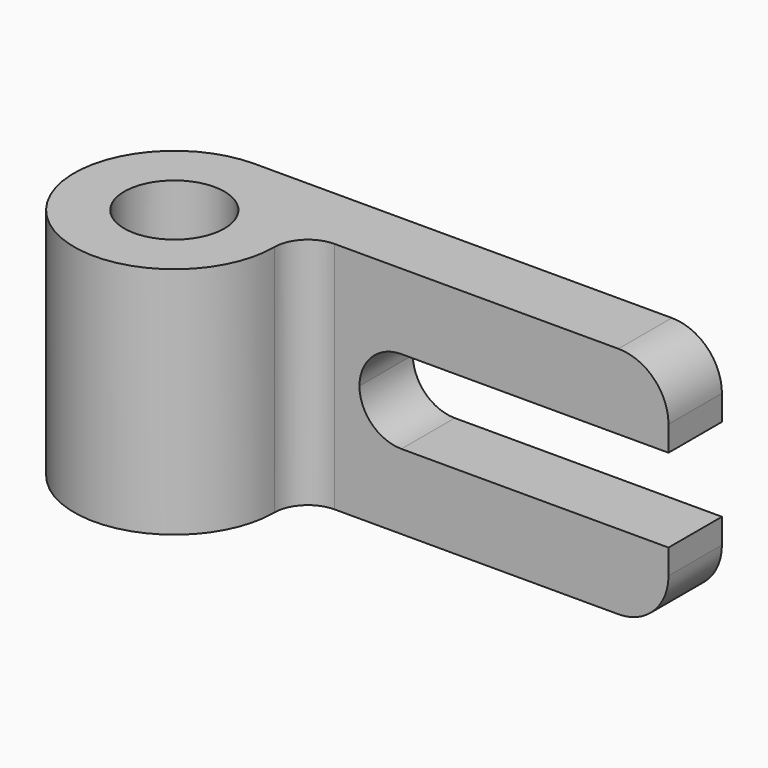
from build123d import *

# Parameters (mm, degrees)
F0_R        = 9.525
F1_DEPTH    = 44.45
F2_T1_DEPTH = 44.45
F3_R        = 9.525
F4_W        = 58.7756
F4_H        = 15.875
F5_DEPTH    = 25.4
F6_T1_DEPTH = 12.7


# Not quite as in the source:
# - a fillet or chamfer that OpenCascade refuses, or shapes differently, is made with other operations: its cross-section is extruded or revolved along the edge and cut away or added


with BuildPart() as f1:
    # F0 (on Top) → F1 (new body)
    with BuildSketch(Plane.XY):
        with BuildLine():
            ThreePointArc((0, 19.05), (10.9985226281, 15.5542598667), (17.9605122421, 6.35))
            Line((17.9605122421, 6.35), (88.9, 6.35))
            Line((88.9, 6.35), (88.9, 19.05))
            Line((88.9, 19.05), (0, 19.05))
        make_face()
        with BuildLine():
            ThreePointArc((0, 19.05), (-13.4703841816, -13.4703841816), (19.05, 0))
            ThreePointArc((19.05, 0), (18.7756525614, 3.2213926947), (17.9605122421, 6.35))
            ThreePointArc((17.9605122421, 6.35), (10.9985226281, 15.5542598667), (0, 19.05))
        make_face()
        Circle(F0_R, mode=Mode.SUBTRACT)
    extrude(amount=F1_DEPTH)

    # F2: fillet of radius 6.35 on 1 edges, made by hand

    # F2_s2 → F2_t1 (join)
    with BuildSketch(Plane.XY):
        with BuildLine():
            ThreePointArc((25.4, 6.35), (20.9098719395, 4.4901280605), (19.05, 0))
            ThreePointArc((19.05, 0), (18.7756525614, 3.2213926947), (17.9605122421, 6.35))
            Line((17.9605122421, 6.35), (25.4, 6.35))
        make_face()
    extrude(amount=F2_T1_DEPTH)

    # F3
    f3_edges = [f1.edges().sort_by_distance(p)[0] for p in [
        (88.9, 12.7, 44.45),
        (88.9, 12.7, 0),
    ]]
    fillet(f3_edges, radius=F3_R)

    # F4 (on face) → F5 (cut)
    with BuildSketch(Plane.XZ.offset(-6.35)):
        with Locations((59.5122, 22.2023769543)):
            Rectangle(F4_W, F4_H)
    extrude(amount=-F5_DEPTH, mode=Mode.SUBTRACT)

    # F6: fillet of radius 7.9756 on 2 edges, made by hand

    # F6_s2 → F6_t1 (join)
    with BuildSketch(Plane.XZ.offset(-19.05)):
        with BuildLine():
            ThreePointArc((30.1244, 22.1642769543), (32.460399156, 27.8038777983), (38.1, 30.1398769543))
            Line((38.1, 30.1398769543), (30.1244, 30.1398769543))
            Line((30.1244, 30.1398769543), (30.1244, 22.1642769543))
        make_face()
        with BuildLine():
            ThreePointArc((38.1, 14.2648769543), (32.460399156, 16.6008761102), (30.1244, 22.2404769543))
            Line((30.1244, 22.2404769543), (30.1244, 14.2648769543))
            Line((30.1244, 14.2648769543), (38.1, 14.2648769543))
        make_face()
    extrude(amount=F6_T1_DEPTH)


solid = f1.part
